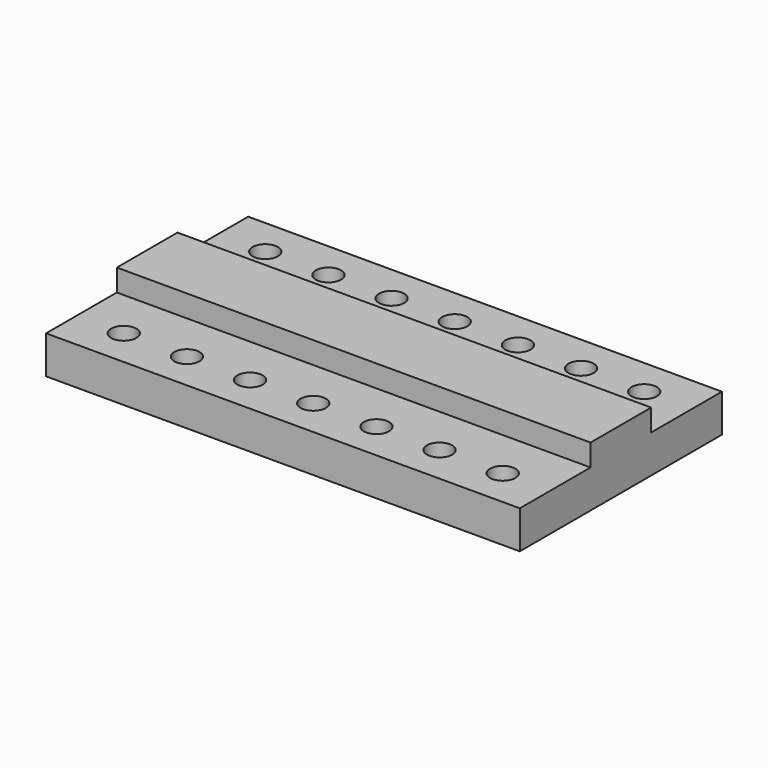
from build123d import *

# Parameters (mm, degrees)
F0_W      = 95.25
F0_H      = 50.8
F1_DEPTH  = 7.62
F2_R      = 2.54
F3_DEPTH  = 7.621
F4_W      = 10.16
F4_H      = 5.08
F5_DEPTH  = 95.251
F8_R      = 1.27
F9_DEPTH  = 27.2604090512
F12_R     = 1.27
F13_DEPTH = 29.4601135768
F15_DEPTH = 95.25
F16_W     = 2.54
F16_H     = 10.16


with BuildPart() as f1:
    # F0 (on Top) → F1 (new body)
    with BuildSketch(Plane.XY):
        Rectangle(F0_W, F0_H)
    extrude(amount=F1_DEPTH)

    # F2 (on face) → F3 (cut, through all)
    with BuildSketch(Plane.XY.offset(7.62)):
        with Locations((-38.1, 17.78)):
            Circle(F2_R)
        with Locations((-38.1, -17.78)):
            Circle(F2_R)
        with Locations((-25.4, 17.78)):
            Circle(F2_R)
        with Locations((-25.4, -17.78)):
            Circle(F2_R)
        with Locations((-12.7, 17.78)):
            Circle(F2_R)
        with Locations((-12.7, -17.78)):
            Circle(F2_R)
        with Locations((0, 17.78)):
            Circle(F2_R)
        with Locations((0, -17.78)):
            Circle(F2_R)
        with Locations((12.7, 17.78)):
            Circle(F2_R)
        with Locations((12.7, -17.78)):
            Circle(F2_R)
        with Locations((25.4, 17.78)):
            Circle(F2_R)
        with Locations((25.4, -17.78)):
            Circle(F2_R)
        with Locations((38.1, 17.78)):
            Circle(F2_R)
        with Locations((38.1, -17.78)):
            Circle(F2_R)
    extrude(amount=-F3_DEPTH, mode=Mode.SUBTRACT)

    # F4 (on face) → F5 (cut, through all)
    with BuildSketch(Plane.YZ.offset(47.625)):
        with Locations((0, 7.62)):
            Rectangle(F4_W, F4_H)
    extrude(amount=-F5_DEPTH, mode=Mode.SUBTRACT)

    # F8 (on face) → F9 (cut, through all)
    with BuildSketch(Plane(origin=(0, -7.2797045256, 12.6088181024), x_dir=(1, 0, 0), z_dir=(0, 0.5, -0.8660254038))):
        with Locations((-42.545, -8.2094090512)):
            Circle(F8_R)
        with Locations((-32.385, -8.2094090512)):
            Circle(F8_R)
        with Locations((-22.225, -8.2094090512)):
            Circle(F8_R)
        with Locations((-12.065, -8.2094090512)):
            Circle(F8_R)
        with Locations((-1.905, -8.2094090512)):
            Circle(F8_R)
        with Locations((8.255, -8.2094090512)):
            Circle(F8_R)
        with Locations((18.415, -8.2094090512)):
            Circle(F8_R)
        with Locations((28.575, -8.2094090512)):
            Circle(F8_R)
        with Locations((38.735, -8.2094090512)):
            Circle(F8_R)
        with Locations((48.895, -8.2094090512)):
            Circle(F8_R)
    extrude(amount=F9_DEPTH, mode=Mode.SUBTRACT)

    # F12 (on face) → F13 (cut, through all)
    with BuildSketch(Plane(origin=(0, 8.3795567884, 14.5138181024), x_dir=(1, 0, 0), z_dir=(0, -0.5, -0.8660254038))):
        with Locations((42.545, 8.2094090512)):
            Circle(F12_R)
        with Locations((32.385, 8.2094090512)):
            Circle(F12_R)
        with Locations((22.225, 8.2094090512)):
            Circle(F12_R)
        with Locations((12.065, 8.2094090512)):
            Circle(F12_R)
        with Locations((1.905, 8.2094090512)):
            Circle(F12_R)
        with Locations((-8.255, 8.2094090512)):
            Circle(F12_R)
        with Locations((-18.415, 8.2094090512)):
            Circle(F12_R)
        with Locations((-28.575, 8.2094090512)):
            Circle(F12_R)
        with Locations((-38.735, 8.2094090512)):
            Circle(F12_R)
        with Locations((-48.895, 8.2094090512)):
            Circle(F12_R)
    extrude(amount=F13_DEPTH, mode=Mode.SUBTRACT)

    # F14 (on face) → F15 (join, through all)
    with BuildSketch(Plane.YZ.offset(47.625)):
        Polygon((-7.62, 12.0324302436), (-7.62, 7.62), (-5.08, 7.62), (0, 10.7624302436), (5.08, 7.62), (7.62, 7.62), (7.62, 12.0324302436), align=None)
    extrude(amount=-F15_DEPTH)

    # F16 (on face) → F17 (join, up to the next surface of F1)
    with BuildSketch(Plane.XY.offset(5.08)):
        with Locations((46.355, 0)):
            Rectangle(F16_W, F16_H)
    extrude(until=Until.NEXT)


solid = f1.part
